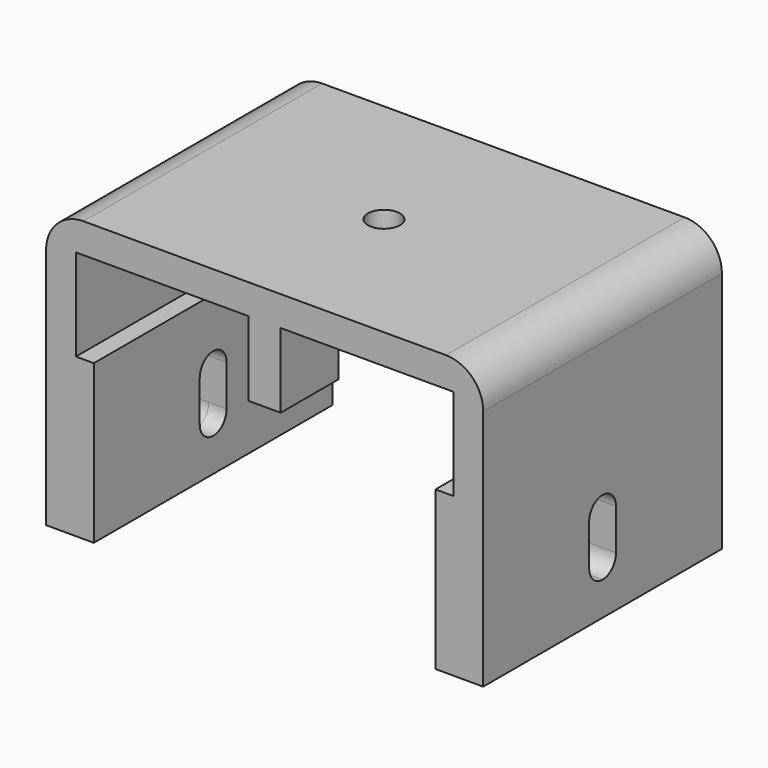
from build123d import *

# Parameters (mm, degrees)
F1_DEPTH  = 40
F2_R      = 5
F3_R      = 2.15
F4_DEPTH  = 25
F5_W      = 4.5
F5_H      = 10
F6_DEPTH  = 58.601
F7_R      = 2.24999
F8_W      = 40
F8_H      = 21.2
F9_DEPTH  = 2.4
F10_W     = 40
F10_H     = 21.2
F11_DEPTH = 2.4
F12_W     = 4.3
F12_H     = 9.6518629789
F13_DEPTH = 10


# Not quite as in the source:
# - a fillet or chamfer is up to 0.001 mm smaller than in the source, because OpenCascade refuses the exact size


with BuildPart() as f1:
    # F0 (on Front) → F1 (new body)
    with BuildSketch(Plane.XZ):
        Polygon((25.3, -18.75), (29.3, -18.75), (29.3, 18.75), (-29.3, 18.75), (-29.3, -18.75), (-25.3, -18.75), (-25.3, 14.75), (25.3, 14.75), align=None)
    extrude(amount=F1_DEPTH)

    # F2
    f2_edges = [f1.edges().sort_by_distance(p)[0] for p in [
        (-29.3, -20, 18.75),
        (29.3, -20, 18.75),
    ]]
    fillet(f2_edges, radius=F2_R)

    # F3 (on face) → F4 (cut)
    with BuildSketch(Plane.XY.offset(18.75)):
        with Locations((0, -20)):
            Circle(F3_R)
    extrude(amount=-F4_DEPTH, mode=Mode.SUBTRACT)

    # F5 (on face) → F6 (cut, through all)
    with BuildSketch(Plane.YZ.offset(29.3)):
        with Locations((-20, -9.25)):
            Rectangle(F5_W, F5_H)
    extrude(amount=-F6_DEPTH, mode=Mode.SUBTRACT)

    # F7 (radius 2.25 in the source; OpenCascade refuses exactly that, so slightly less here)
    f7_edges = [f1.edges().sort_by_distance(p)[0] for p in [
        (27.3, -17.75, -4.25),
        (27.3, -22.25, -4.25),
        (27.3, -17.75, -14.25),
        (27.3, -22.25, -14.25),
        (-27.3, -17.75, -4.25),
        (-27.3, -17.75, -14.25),
        (-27.3, -22.25, -4.25),
        (-27.3, -22.25, -14.25),
    ]]
    fillet(f7_edges, radius=F7_R)

    # F8 (on face) → F9 (join)
    with BuildSketch(Plane(origin=(25.3, 0, 0), x_dir=(0, -1, 0), z_dir=(-1, 0, 0))):
        with Locations((20, -8.15)):
            Rectangle(F8_W, F8_H)
        with BuildLine():
            ThreePointArc((17.75, -6.5), (20, -4.25), (22.25, -6.5))
            Line((22.25, -6.5), (22.25, -12))
            ThreePointArc((22.25, -12), (20, -14.25), (17.75, -12))
            Line((17.75, -12), (17.75, -6.5))
        make_face(mode=Mode.SUBTRACT)
    extrude(amount=F9_DEPTH)

    # F10 (on face) → F11 (join)
    with BuildSketch(Plane.YZ.offset(-25.3)):
        with Locations((-20, -8.15)):
            Rectangle(F10_W, F10_H)
        with BuildLine():
            ThreePointArc((-22.25, -6.5), (-20, -4.25), (-17.75, -6.5))
            Line((-17.75, -6.5), (-17.75, -12))
            ThreePointArc((-17.75, -12), (-20, -14.25), (-22.25, -12))
            Line((-22.25, -12), (-22.25, -6.5))
        make_face(mode=Mode.SUBTRACT)
    extrude(amount=F11_DEPTH)

    # F12 (on face) → F13 (join)
    with BuildSketch(Plane(origin=(0, 0, 14.75), x_dir=(1, 0, 0), z_dir=(0, 0, -1))):
        with Locations((0, 35.1740685105)):
            Rectangle(F12_W, F12_H)
    extrude(amount=F13_DEPTH)


solid = f1.part
